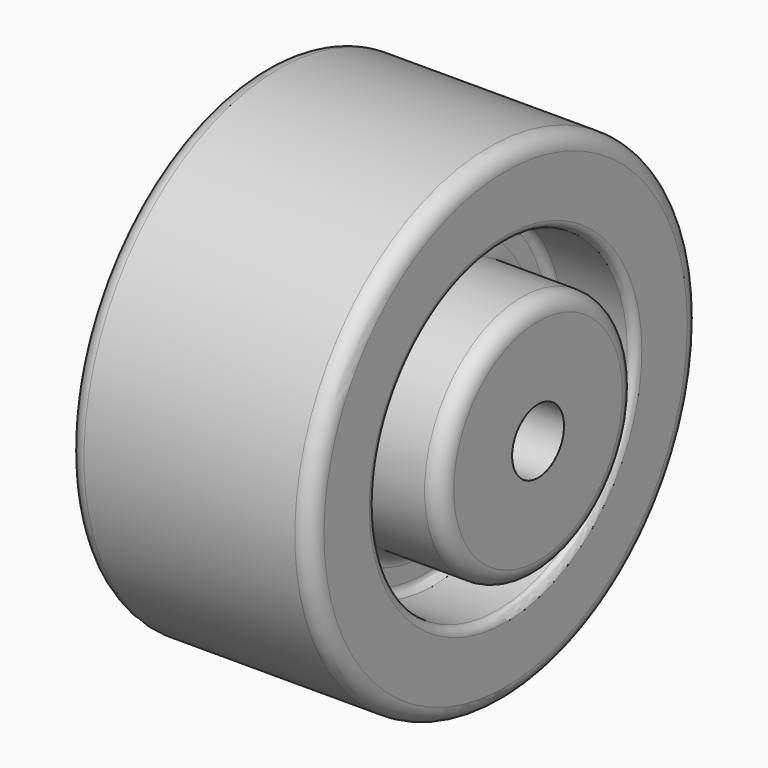
from build123d import *

# Parameters (mm, degrees)
F0_R      = 75
F1_DEPTH  = 75
F2_R      = 5
F3_R      = 50
F4_DEPTH  = 5
F5_R      = 2.49999
F6_R      = 50
F7_DEPTH  = 25
F8_R      = 2.5
F9_R      = 37.5
F9_R_2    = 10
F10_DEPTH = 35
F11_R     = 5


# Not quite as in the source:
# - a fillet or chamfer is up to 0.001 mm smaller than in the source, because OpenCascade refuses the exact size


with BuildPart() as f1:
    # F0 (on Right) → F1 (new body)
    with BuildSketch(Plane.YZ):
        Circle(F0_R)
    extrude(amount=F1_DEPTH)

    # F2
    f2_edges = [f1.edges().sort_by_distance(p)[0] for p in [
        (37.5, 75, 0),
        (0, -75, 0),
        (75, -75, 0),
    ]]
    fillet(f2_edges, radius=F2_R)

    # F3 (on face) → F4 (cut)
    with BuildSketch(Plane(origin=(0, 0, 0), x_dir=(0, -1, 0), z_dir=(-1, 0, 0))):
        Circle(F3_R)
    extrude(amount=-F4_DEPTH, mode=Mode.SUBTRACT)

    # F5 (radius 2.5 in the source; OpenCascade refuses exactly that, so slightly less here)
    f5_edges = [f1.edges().sort_by_distance(p)[0] for p in [
        (5, 50, 0),
        (0, 50, 0),
    ]]
    fillet(f5_edges, radius=F5_R)

    # F6 (on face) → F7 (cut)
    with BuildSketch(Plane.YZ.offset(75)):
        Circle(F6_R)
    extrude(amount=-F7_DEPTH, mode=Mode.SUBTRACT)

    # F8
    f8_edges = [f1.edges().sort_by_distance(p)[0] for p in [
        (50, -50, 0),
        (75, -50, 0),
    ]]
    fillet(f8_edges, radius=F8_R)

    # F9 (on face) → F10 (join)
    with BuildSketch(Plane.YZ.offset(50)):
        Circle(F9_R)
        Circle(F9_R_2, mode=Mode.SUBTRACT)
    extrude(amount=F10_DEPTH)

    # F11
    f11_edges = [f1.edges().sort_by_distance(p)[0] for p in [
        (50, -37.5, 0),
        (85, -37.5, 0),
    ]]
    fillet(f11_edges, radius=F11_R)


solid = f1.part
